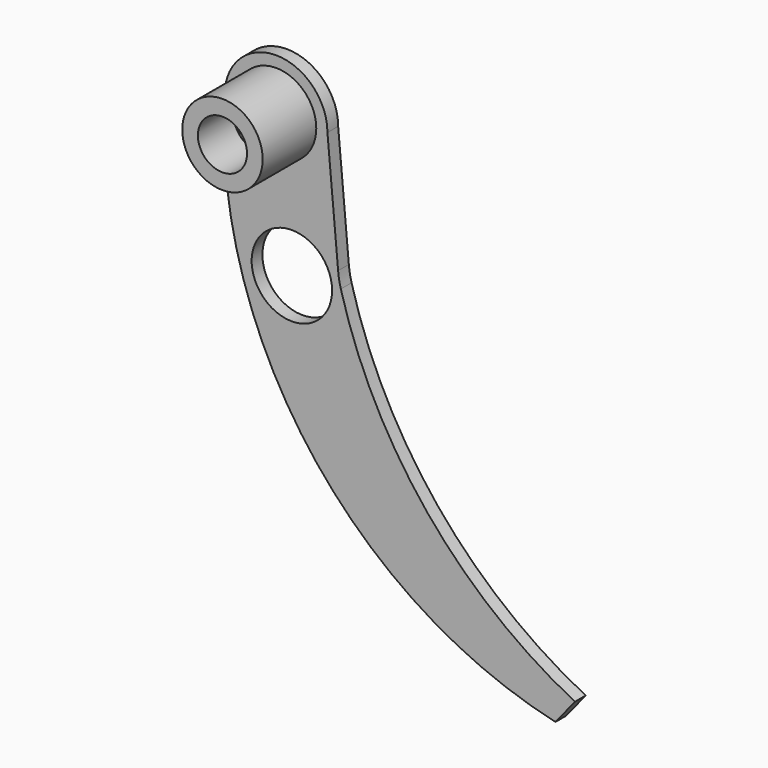
from build123d import *

# Parameters (mm, degrees)
F0_R     = 45
F1_DEPTH = 15
F0_R_2   = 27.5
F0_R_3   = 25
F2_DEPTH = 40
F3_DEPTH = 90


# Not quite as in the source:
# - ends of sketch curves that miss each other by under 0.0002 mm in the source are joined


with BuildPart() as f1:
    # F0 (on Front) → F1 (new body)
    with BuildSketch(Plane.XZ):
        with BuildLine():
            ThreePointArc((384.6949439554, 791.790903988), (382.803167543, 800.2488212516), (381.650846946, 808.8387769951))
            Line((381.650846946, 808.8387769951), (369.718198, 941.060787))
            ThreePointArc((369.718198, 941.060787), (311.2324816498, 998.5523373642), (254.7519940599, 939.0896440021))
            ThreePointArc((254.7519940599, 939.0896440021), (348.7062296758, 623.1920986799), (624.9311859905, 443.4188219584))
            Line((624.9311859905, 443.4188219584), (646.703822, 470.414472))
            ThreePointArc((646.703822, 470.414472), (481.4005278043, 603.1398267524), (384.6949439554, 791.790903988))
        make_face()
        with Locations((329.907435, 787.07348)):
            Circle(F0_R, mode=Mode.SUBTRACT)
        with Locations((312.218198, 941.060787)):
            Circle(F0_R, mode=Mode.SUBTRACT)
    extrude(amount=F1_DEPTH)

    # F0 (on Front) → F3 (join)
    with BuildSketch(Plane.XZ):
        with Locations((312.218198, 941.060787)):
            Circle(F0_R)
        with Locations((312.218198, 941.060787)):
            Circle(F0_R_2, mode=Mode.SUBTRACT)
    extrude(amount=F3_DEPTH)


with BuildPart() as f2:
    # F0 (on Front) → F2 (new body)
    with BuildSketch(Plane.XZ):
        with Locations((312.218198, 941.060787)):
            Circle(F0_R_2)
        with Locations((312.218198, 941.060787)):
            Circle(F0_R_3, mode=Mode.SUBTRACT)
    extrude(amount=F2_DEPTH)


solid = Compound([f1.part, f2.part])
